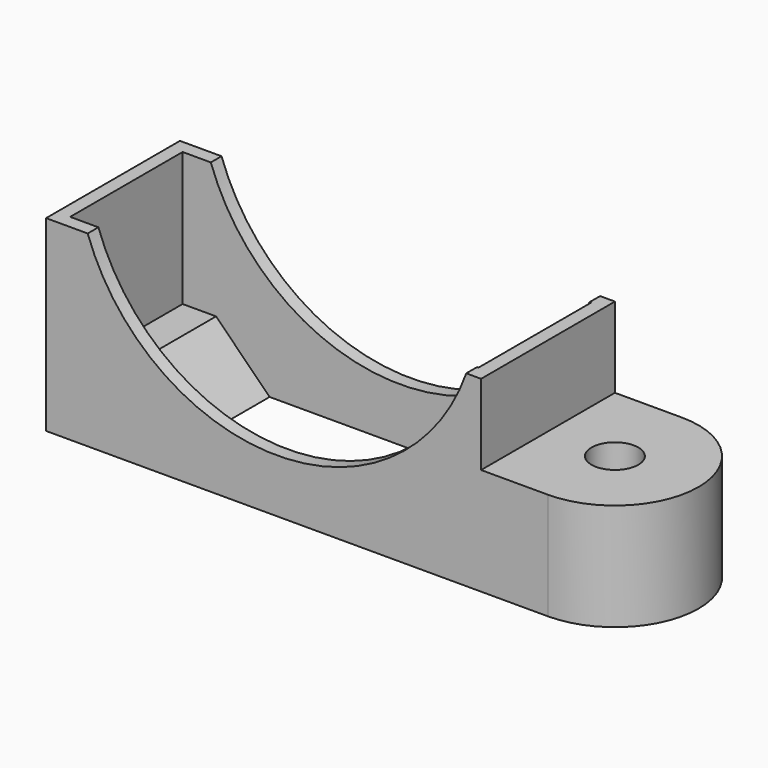
from build123d import *

# Parameters (mm, degrees)
F0_R     = 1.75
F1_DEPTH = 8
F0_W     = 32.5
F0_H     = 12.5
F2_DEPTH = 14
F0_W_2   = 6.5
F0_H_2   = 10.5
F3_DEPTH = 4
F4_SIZE  = 3.99999
F6_DEPTH = 25
F7_R     = 3.75
F7_R_2   = 1.75
F8_DEPTH = 3


# Not quite as in the source:
# - a fillet or chamfer is up to 0.001 mm smaller than in the source, because OpenCascade refuses the exact size


with BuildPart() as f1:
    # F0 (on Top) → F1 (new body)
    with BuildSketch(Plane.XY):
        with BuildLine():
            Line((16.25, 6.25), (16.25, -6.25))
            Line((16.25, -6.25), (21.25, -6.25))
            ThreePointArc((21.25, -6.25), (27.5, 0), (21.25, 6.25))
            Line((21.25, 6.25), (16.25, 6.25))
        make_face()
        with Locations((21.25, 0)):
            Circle(F0_R, mode=Mode.SUBTRACT)
    extrude(amount=F1_DEPTH)

    # F0 (on Top) → F2 (join)
    with BuildSketch(Plane.XY):
        Rectangle(F0_W, F0_H)
        Polygon((15.25, 5.25), (15.25, -5.25), (8.75, -5.25), (-8.75, -5.25), (-15.25, -5.25), (-15.25, 5.25), (-8.75, 5.25), (8.75, 5.25), align=None, mode=Mode.SUBTRACT)
    extrude(amount=F2_DEPTH)

    # F0 (on Top) → F3 (join)
    with BuildSketch(Plane.XY):
        with Locations((12, 0)):
            Rectangle(F0_W_2, F0_H_2)
        with Locations((-12, 0)):
            Rectangle(F0_W_2, F0_H_2)
    extrude(amount=F3_DEPTH)

    # F4 (size 4 in the source; OpenCascade refuses exactly that, so slightly less here)
    f4_edges = [f1.edges().sort_by_distance(p)[0] for p in [
        (-8.75, 0, 4),
        (8.75, 0, 0),
    ]]
    chamfer(f4_edges, length=F4_SIZE)

    # F5 (on face) → F6 (cut)
    with BuildSketch(Plane.XZ.offset(6.25)):
        with BuildLine():
            Line((15.1421356237, 14), (-13.1421356237, 14))
            ThreePointArc((-13.1421356237, 14), (1, 4), (15.1421356237, 14))
        make_face()
    extrude(amount=-F6_DEPTH, mode=Mode.SUBTRACT)

    # F7 (on face) → F8 (cut)
    with BuildSketch(Plane.XY):
        with Locations((21.25, 0)):
            Circle(F7_R)
        with Locations((21.25, 0)):
            Circle(F7_R_2, mode=Mode.SUBTRACT)
    extrude(amount=F8_DEPTH, mode=Mode.SUBTRACT)


solid = f1.part
